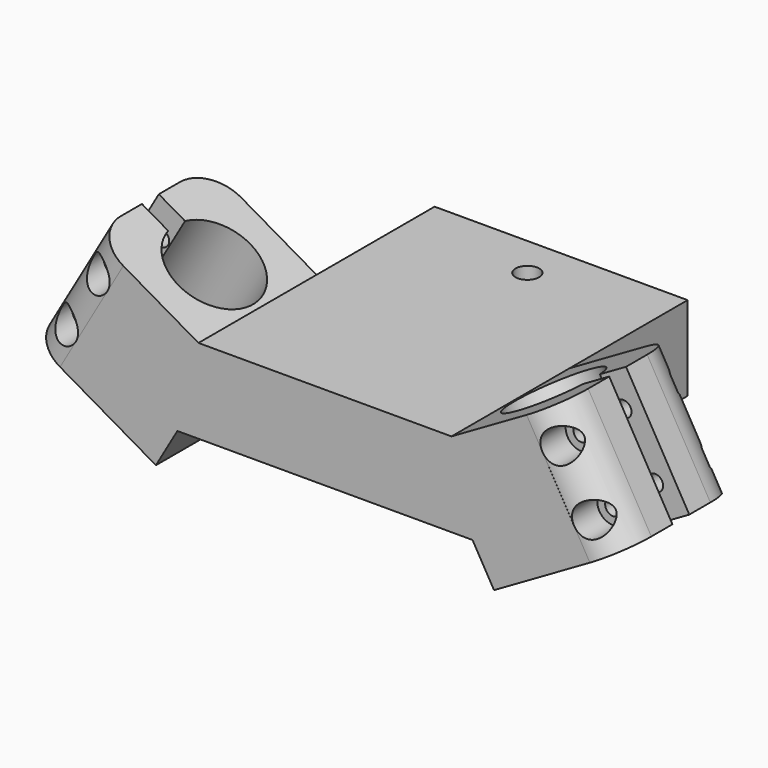
from build123d import *

# Parameters (mm, degrees)
F1_DEPTH       = 44.45
F2_R           = 13.49375
F3_DEPTH       = 38.1
F4_W           = 6.35
F4_H           = 38.1
F5_DEPTH       = 9.1110976343
F7_D           = 4.7625
F7_CBORE_D     = 9.525
F7_CBORE_DEPTH = 9.525
F8_R           = 2.38125
F9_DEPTH       = 9.525
F10_T1_DEPTH   = 93.6625
F11_W          = 76.2
F11_H          = 25.4
F12_DEPTH      = 44.45
F14_D          = 7.14375
F15_T1_DEPTH   = 93.6625


# Not quite as in the source:
# - a fillet or chamfer that OpenCascade refuses, or shapes differently, is made with other operations: its cross-section is extruded or revolved along the edge and cut away or added
# - a pattern or mirror of a feature is missing from the dataset's text; its kind, count and spacing are read off the source's solid


with BuildPart() as f1:
    # F0 (on Front) → F1 (new body)
    with BuildSketch(Plane.XZ):
        Polygon((38.1, 0), (0, 0), (-38.1, 0), (-70.3588065702, 18.624630657), (-89.4088065702, -14.3709372272), (-50.9139773719, -36.5959372272), (-44.45, -25.4), (0, -25.4), (44.45, -25.4), (50.9139773719, -36.5959372272), (89.4088065702, -14.3709372272), (70.3588065702, 18.624630657), align=None)
    extrude(amount=F1_DEPTH)

    # F2 (on face) → F3 (cut, through all)
    with BuildSketch(Plane(origin=(28.575, 0, -49.4933518263), x_dir=(0.8660254038, 0, 0.5), z_dir=(0.5, 0, -0.8660254038))):
        with Locations((48.0198291982, 22.225)):
            Circle(F2_R)
    f3 = extrude(amount=-F3_DEPTH, mode=Mode.SUBTRACT)

    # F3_copies: F3 across plane
    add(f3.mirror(Plane(origin=(0, 0, 0), x_dir=(0, 0, -1), z_dir=(-1, 0, 0))), mode=Mode.SUBTRACT)

    # F4 (on face) → F5 (cut, through all)
    with BuildSketch(Plane(origin=(60.8338065702, 0, 35.1224145991), x_dir=(0, 1, 0), z_dir=(0.8660254038, 0, 0.5))):
        with Locations((-22.225, -38.1)):
            Rectangle(F4_W, F4_H)
    f5 = extrude(amount=-F5_DEPTH, mode=Mode.SUBTRACT)

    # F5_copies: F5 across plane
    add(f5.mirror(Plane(origin=(0, 0, 0), x_dir=(0, 0, -1), z_dir=(-1, 0, 0))), mode=Mode.SUBTRACT)

    # F7 (through all)
    with Locations(Plane.XZ.offset(44.45)):
        with Locations((69.6220452561, 7.200738686), (79.1470452561, -9.2970452561)):
            f7 = CounterBoreHole(F7_D / 2, F7_CBORE_D / 2, F7_CBORE_DEPTH)

    # F7_copies: F7 across plane
    add(f7.mirror(Plane(origin=(0, 0, 0), x_dir=(0, 0, -1), z_dir=(-1, 0, 0))), mode=Mode.SUBTRACT)

    # F8 (on face) → F9 (cut)
    with BuildSketch(Plane(origin=(0, 0, 0), x_dir=(-1, 0, 0), z_dir=(0, 1, 0))):
        Polygon((-64.5810557183, 7.200738686), (-67.1015504872, 11.566363686), (-72.1425400251, 11.566363686), (-74.663034794, 7.200738686), (-72.1425400251, 2.835113686), (-67.1015504872, 2.835113686), align=None)
        with Locations((-69.6220452561, 7.200738686)):
            Circle(F8_R, mode=Mode.SUBTRACT)
        Polygon((-76.6265504872, -13.6626702561), (-74.1060557183, -9.2970452561), (-76.6265504872, -4.9314202561), (-81.6675400251, -4.9314202561), (-84.188034794, -9.2970452561), (-81.6675400251, -13.6626702561), align=None)
        with Locations((-79.1470452561, -9.2970452561)):
            Circle(F8_R, mode=Mode.SUBTRACT)
    f9 = extrude(amount=-F9_DEPTH, mode=Mode.SUBTRACT)

    # F9_copies: F9 across plane
    add(f9.mirror(Plane(origin=(0, 0, 0), x_dir=(0, 0, -1), z_dir=(-1, 0, 0))), mode=Mode.SUBTRACT)

    # F10: fillet of radius 11.1125 on 2 edges, made by hand

    # F10_s2 → F10_t1 (cut)
    with BuildSketch(Plane(origin=(42.465625, 0, -73.5526200752), x_dir=(0, 1, 0), z_dir=(-0.5, 0, 0.8660254038))):
        with BuildLine():
            ThreePointArc((-44.45, -59.1323291982), (-41.1952241059, -66.9900533042), (-33.3375, -70.2448291982))
            Line((-33.3375, -70.2448291982), (-44.45, -70.2448291982))
            Line((-44.45, -70.2448291982), (-44.45, -59.1323291982))
        make_face()
        with BuildLine():
            ThreePointArc((-11.1125, -70.2448291982), (-3.2547758941, -66.9900533042), (0, -59.1323291982))
            Line((0, -59.1323291982), (0, -70.2448291982))
            Line((0, -70.2448291982), (-11.1125, -70.2448291982))
        make_face()
    extrude(amount=F10_T1_DEPTH, mode=Mode.SUBTRACT)

    # F11 (on face) → F12 (join)
    with BuildSketch(Plane(origin=(0, 0, 0), x_dir=(-1, 0, 0), z_dir=(0, 1, 0))):
        with Locations((0, -12.7)):
            Rectangle(F11_W, F11_H)
    extrude(amount=F12_DEPTH)

    # F14 (through all)
    with Locations(Plane.XY):
        with Locations((0, 31.75)):
            Hole(F14_D / 2)

    # F15: fillet of radius 11.1125 on 2 edges, made by hand

    # F15_s2 → F15_t1 (cut)
    with BuildSketch(Plane(origin=(4.365625, 0, 7.5614843068), x_dir=(0, 1, 0), z_dir=(-0.5, 0, -0.8660254038))):
        with BuildLine():
            ThreePointArc((0, -59.1323291982), (-3.2547758941, -66.9900533042), (-11.1125, -70.2448291982))
            Line((-11.1125, -70.2448291982), (0, -70.2448291982))
            Line((0, -70.2448291982), (0, -59.1323291982))
        make_face()
        with BuildLine():
            ThreePointArc((-44.45, -59.1323291982), (-41.1952241059, -66.9900533042), (-33.3375, -70.2448291982))
            Line((-33.3375, -70.2448291982), (-44.45, -70.2448291982))
            Line((-44.45, -70.2448291982), (-44.45, -59.1323291982))
        make_face()
    extrude(amount=F15_T1_DEPTH, mode=Mode.SUBTRACT)


solid = f1.part
